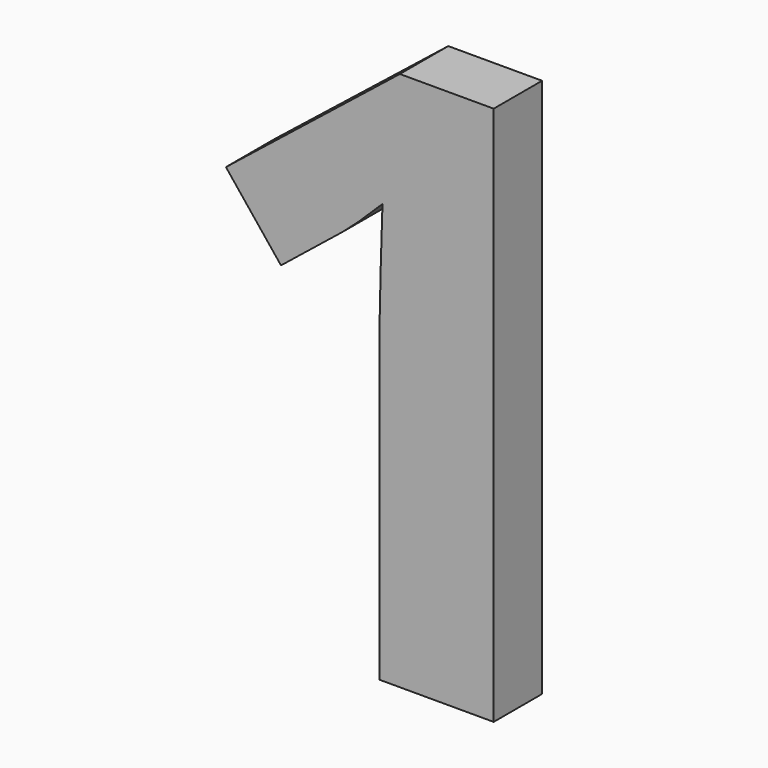
from build123d import *

# Parameters (mm, degrees)
F0_TEXT_SIZE = 62.5
F1_DEPTH     = 5


# Not quite as in the source:
# - Text() gives the source's letters only with a copy of the font that has no kerning and outlines rounded to 1/6400 em; it was checked with that copy


with BuildPart() as f1:
    # F0 (on Front) → F1 (new body)
    with BuildSketch(Plane.XZ):
        with Locations((-54.1507152475, 9.5813388195)):
            Text('1', F0_TEXT_SIZE, font='Open Sans', font_style=FontStyle.BOLD, text_align=(TextAlign.LEFT, TextAlign.BOTTOM))
    extrude(amount=F1_DEPTH)


solid = f1.part
